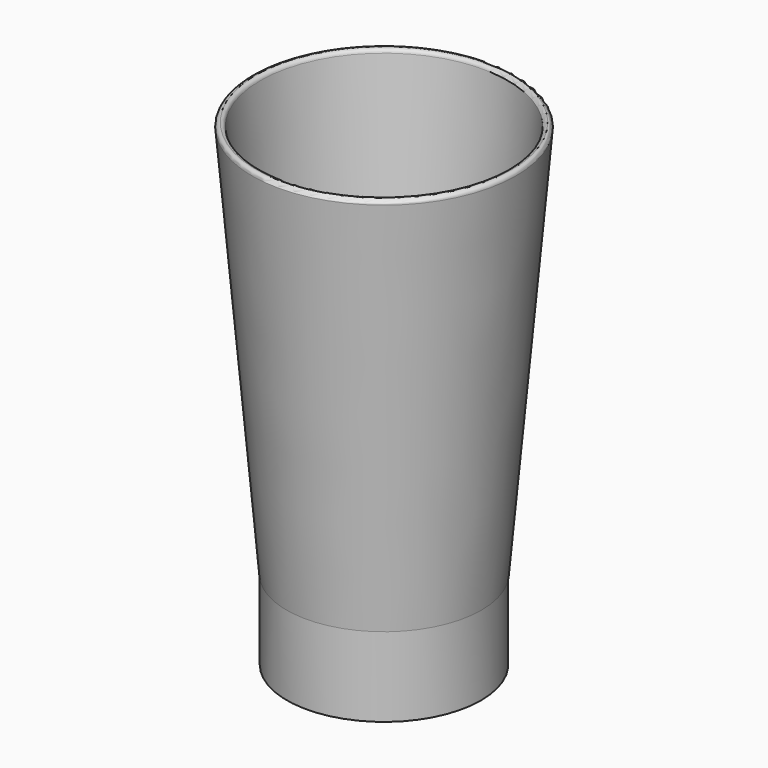
from build123d import *

# Parameters (mm, degrees)
F0_R     = 44.45
F1_DEPTH = 63.5
F3_T     = -2.54
F4_R     = 1.26999
F5_R     = 30.988
F6_DEPTH = 25.4


# Not quite as in the source:
# - a fillet or chamfer that OpenCascade refuses, or shapes differently, is made with other operations: its cross-section is extruded or revolved along the edge and cut away or added
# - a fillet or chamfer is up to 0.001 mm smaller than in the source, because OpenCascade refuses the exact size


with BuildPart() as f1:
    # F0 (on Top) → F1 (new body, symmetric)
    with BuildSketch(Plane.XY):
        Circle(F0_R)
    extrude(amount=F1_DEPTH, both=True)

    # F2: chamfer of 152.4 x 13.3332723214 on 1 edges, made by hand

    # F2_s1 → F2_t2 (revolve, cut)
    with BuildSketch(Plane.XZ):
        Polygon((44.45, 88.9), (31.1167276786, -63.5), (44.45, -63.5), align=None)
    revolve(axis=Axis((0, 0, -63.5), (0, 0, 1)), mode=Mode.SUBTRACT)

    # F3
    f3_openings = [f1.faces().sort_by_distance(p)[0] for p in [
        (0, 0, 63.5),
    ]]
    offset(amount=F3_T, openings=f3_openings)

    # F4 (radius 1.27 in the source; OpenCascade refuses exactly that, so slightly less here)
    f4_edges = [f1.edges().sort_by_distance(p)[0] for p in [
        (-42.227788, 0, 63.5),
        (-39.678086, 0, 63.5),
    ]]
    fillet(f4_edges, radius=F4_R)

    # F5 (on face) → F6 (join)
    with BuildSketch(Plane(origin=(0, 0, -63.5), x_dir=(1, 0, 0), z_dir=(0, 0, -1))):
        Circle(F5_R)
    extrude(amount=F6_DEPTH)


solid = f1.part
